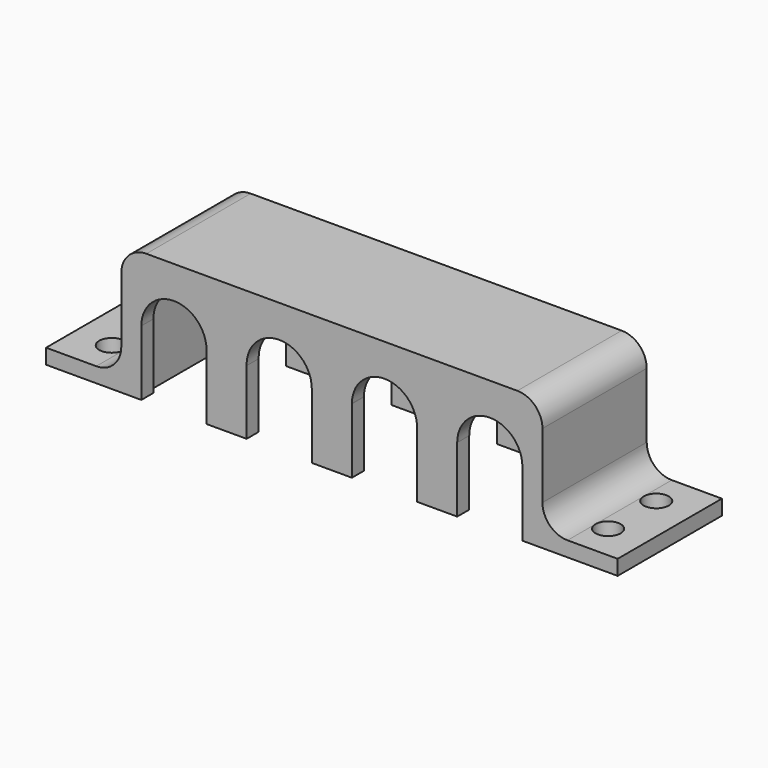
from build123d import *

# Parameters (mm, degrees)
F1_W          = 84
F1_H          = 26
F2_DEPTH      = 13
F2_DEPTH_BACK = 13
F3_T          = -3
F5_W          = 15
F5_H          = 26
F5_R          = 2.5
F5_W_2        = 84
F5_W_3        = 78
F5_H_2        = 20
F6_DEPTH      = 3
F7_R          = 4.99999
F9_DEPTH      = 5
F10_DEPTH     = 25


# Not quite as in the source:
# - a fillet or chamfer is up to 0.001 mm smaller than in the source, because OpenCascade refuses the exact size


with BuildPart() as f2:
    # F1 (on Top) → F2 (new body, two sides)
    with BuildSketch(Plane.XY) as f2_sk:
        with Locations((0, 13)):
            Rectangle(F1_W, F1_H)
    extrude(amount=F2_DEPTH)
    extrude(f2_sk.sketch, amount=-F2_DEPTH_BACK)

    # F3
    f3_openings = [f2.faces().sort_by_distance(p)[0] for p in [
        (0, 13, -13),
    ]]
    offset(amount=F3_T, openings=f3_openings)

    # F5 (on face) → F6 (join)
    with BuildSketch(Plane(origin=(0, 0, -13), x_dir=(1, 0, 0), z_dir=(0, 0, -1))):
        with Locations((-49.5, -13)):
            Rectangle(F5_W, F5_H)
        with Locations((-49.5, -19)):
            Circle(F5_R, mode=Mode.SUBTRACT)
        with Locations((-49.5, -7)):
            Circle(F5_R, mode=Mode.SUBTRACT)
        with Locations((0, -13)):
            Rectangle(F5_W_2, F5_H)
        with Locations((0, -13)):
            Rectangle(F5_W_3, F5_H_2, mode=Mode.SUBTRACT)
        with Locations((49.5, -13)):
            Rectangle(F5_W, F5_H)
        with Locations((49.5, -19)):
            Circle(F5_R, mode=Mode.SUBTRACT)
        with Locations((49.5, -7)):
            Circle(F5_R, mode=Mode.SUBTRACT)
    extrude(amount=-F6_DEPTH)

    # F7 (radius 5 in the source; OpenCascade refuses exactly that, so slightly less here)
    f7_edges = [f2.edges().sort_by_distance(p)[0] for p in [
        (-42, 13, 13),
        (42, 13, 13),
        (-42, 13, -10),
        (42, 13, -10),
        (0, 23, 10),
        (0, 3, 10),
        (-39, 13, 10),
        (39, 13, 10),
    ]]
    fillet(f7_edges, radius=F7_R)

    # F8 (on face) → F9 (cut)
    with BuildSketch(Plane.XZ):
        with BuildLine():
            Line((-25, -11), (-25, 0))
            ThreePointArc((-25, 0), (-31.5, 6.5), (-38, 0))
            Line((-38, 0), (-38, -11))
            Line((-38, -11), (-38, -13))
            Line((-38, -13), (-25, -13))
            Line((-25, -13), (-25, -11))
        make_face()
        with BuildLine():
            Line((-4.0000936475, -11), (-4.0000936475, -0.0348913798))
            ThreePointArc((-4.0000936475, -0.0348913798), (-4, 0), (-4.0000936475, 0.0348913798))
            ThreePointArc((-4.0000936475, 0.0348913798), (-10.5909716955, 6.499363365), (-16.9983365331, -0.1470452389))
            Line((-16.9983365331, -0.1470452389), (-16.9983365331, -10.9773843356))
            Line((-16.9983365331, -10.9773843356), (-16.9983365331, -13))
            Line((-16.9983365331, -13), (-4.0000936475, -13))
            Line((-4.0000936475, -13), (-4.0000936475, -11))
        make_face()
        with BuildLine():
            ThreePointArc((4.0000936475, 0.0348913798), (4, 0), (4.0000936475, -0.0348913798))
            Line((4.0000936475, -0.0348913798), (4.0000936475, -11))
            Line((4.0000936475, -11), (4.0000936475, -13))
            Line((4.0000936475, -13), (16.9983365331, -13))
            Line((16.9983365331, -13), (16.9983365331, -10.9773843356))
            Line((16.9983365331, -10.9773843356), (16.9983365331, -0.1470452389))
            ThreePointArc((16.9983365331, -0.1470452389), (10.5909716955, 6.499363365), (4.0000936475, 0.0348913798))
        make_face()
        with BuildLine():
            ThreePointArc((38, 0), (31.5, 6.5), (25, 0))
            Line((25, 0), (25, -11))
            Line((25, -11), (25, -13))
            Line((25, -13), (38, -13))
            Line((38, -13), (38, -11))
            Line((38, -11), (38, 0))
        make_face()
    extrude(amount=-F9_DEPTH, mode=Mode.SUBTRACT)

    # F4 (on face) → F10 (cut)
    with BuildSketch(Plane(origin=(0, 26, 0), x_dir=(-1, 0, 0), z_dir=(0, 1, 0))):
        with BuildLine():
            Line((-6.5, -13), (-6.5, 0))
            ThreePointArc((-6.5, 0), (-10.5, 4), (-14.5, 0))
            Line((-14.5, 0), (-14.5, -13))
            Line((-14.5, -13), (-6.5, -13))
        make_face()
        with BuildLine():
            Line((-27.5, -13), (-27.5, 0))
            ThreePointArc((-27.5, 0), (-31.5, 4), (-35.5, 0))
            Line((-35.5, 0), (-35.5, -13))
            Line((-35.5, -13), (-27.5, -13))
        make_face()
        with BuildLine():
            ThreePointArc((14.5, 0), (10.5, 4), (6.5, 0))
            Line((6.5, 0), (6.5, -13))
            Line((6.5, -13), (14.5, -13))
            Line((14.5, -13), (14.5, 0))
        make_face()
        with BuildLine():
            ThreePointArc((35.5, 0), (31.5, 4), (27.5, 0))
            Line((27.5, 0), (27.5, -13))
            Line((27.5, -13), (35.5, -13))
            Line((35.5, -13), (35.5, 0))
        make_face()
    extrude(amount=-F10_DEPTH, mode=Mode.SUBTRACT)


solid = f2.part
